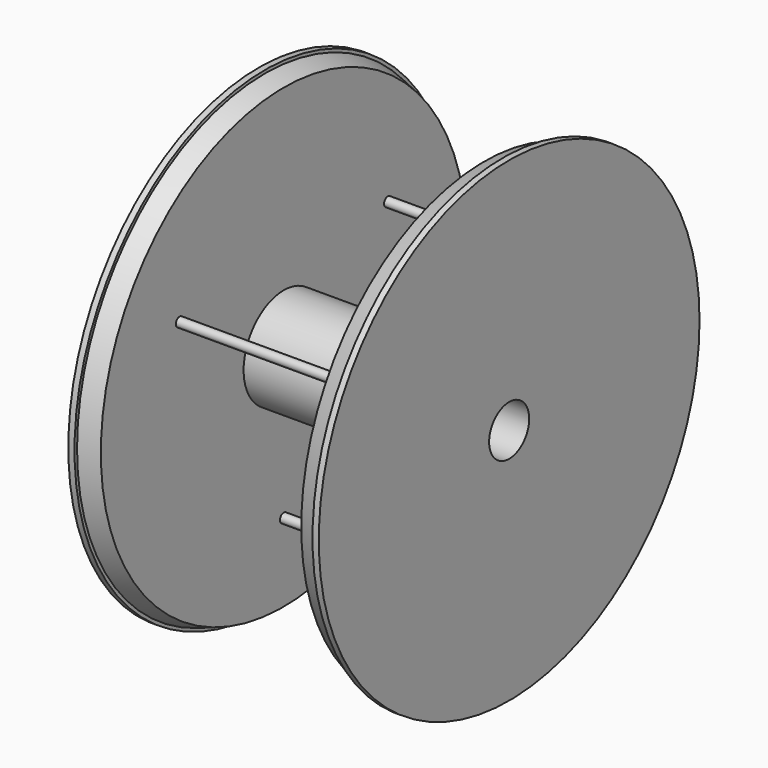
from build123d import *

# Parameters (mm, degrees)
F0_R      = 120.65
F1_DEPTH  = 3.175
F2_R      = 119.0625
F3_DEPTH  = 9.525
F4_SIZE2  = 9.52499
F4_SIZE   = 3.17499
F5_R      = 2.38125
F6_DEPTH  = 101.6
F7_R      = 119.0625
F8_DEPTH  = 9.525
F9_R      = 120.65
F10_DEPTH = 3.175
F11_SIZE2 = 3.17499
F11_SIZE  = 9.52499
F12_R     = 12.7
F13_DEPTH = 127.001


# Not quite as in the source:
# - a fillet or chamfer is up to 0.001 mm smaller than in the source, because OpenCascade refuses the exact size


with BuildPart() as f1:
    # F0 (on Right) → F1 (new body)
    with BuildSketch(Plane.YZ):
        Circle(F0_R)
    extrude(amount=F1_DEPTH)

    # F2 (on face) → F3 (join)
    with BuildSketch(Plane.YZ.offset(3.175)):
        Circle(F2_R)
    extrude(amount=F3_DEPTH)

    # F4 (size 3.175 and 9.525 in the source; OpenCascade refuses exactly that, so slightly less here)
    f4_edges = [f1.edges().sort_by_distance(p)[0] for p in [
        (12.7, -119.0625, 0),
    ]]
    f4_side = f1.faces().sort_by_distance((12.7, 0, 0))[0]
    chamfer(f4_edges, length=F4_SIZE, length2=F4_SIZE2, reference=f4_side)

    # F5 (on face) → F6 (join)
    with BuildSketch(Plane.YZ.offset(12.7)):
        with BuildLine():
            ThreePointArc((21.1539941395, 14.0594641416), (-24.3153393061, -7.3433149482), (25.4, 0))
            ThreePointArc((25.4, 0), (24.3153393061, 7.3433149482), (21.1539941395, 14.0594641416))
        make_face()
        with Locations((0, -76.2)):
            Circle(F5_R)
        with Locations((65.9911357684, 38.1)):
            Circle(F5_R)
        with Locations((-65.9911357684, 38.1)):
            Circle(F5_R)
    extrude(amount=F6_DEPTH)

    # F7 (on face) → F8 (join)
    with BuildSketch(Plane.YZ.offset(114.3)):
        Circle(F7_R)
    extrude(amount=F8_DEPTH)

    # F9 (on face) → F10 (join)
    with BuildSketch(Plane.YZ.offset(123.825)):
        Circle(F9_R)
    extrude(amount=F10_DEPTH)

    # F11 (size 9.525 and 3.175 in the source; OpenCascade refuses exactly that, so slightly less here)
    f11_edges = [f1.edges().sort_by_distance(p)[0] for p in [
        (114.3, -119.0625, 0),
    ]]
    f11_side = f1.faces().sort_by_distance((119.0625, -119.0625, 0))[0]
    chamfer(f11_edges, length=F11_SIZE, length2=F11_SIZE2, reference=f11_side)

    # F12 (on face) → F13 (cut, through all)
    with BuildSketch(Plane.YZ.offset(127)):
        Circle(F12_R)
    extrude(amount=-F13_DEPTH, mode=Mode.SUBTRACT)


solid = f1.part
